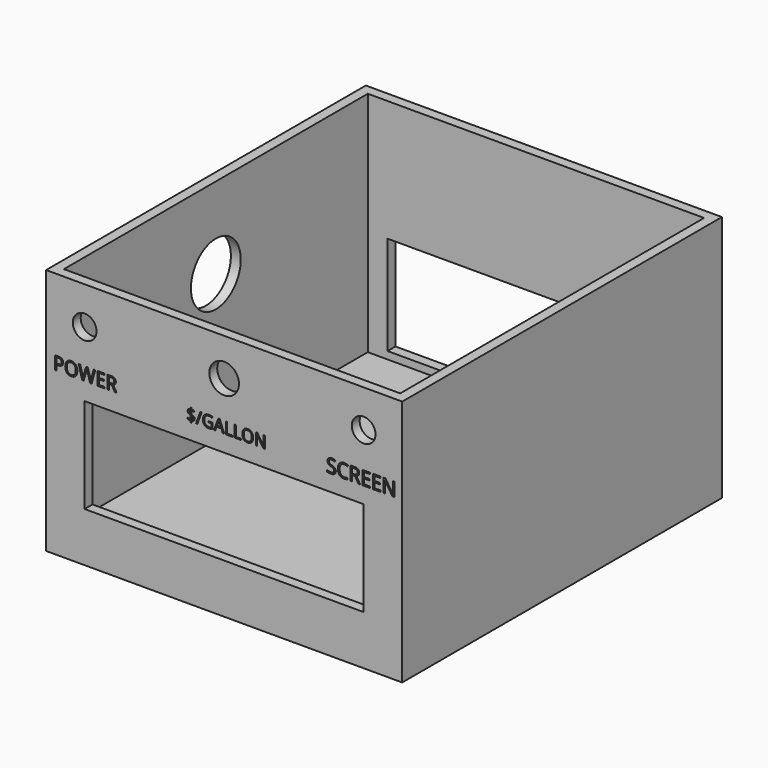
from build123d import *

# Parameters (mm, degrees)
F0_W          = 91.44
F0_H          = 102.616
F1_DEPTH      = 63.5
F2_W          = 86.36
F2_H          = 97.536
F3_DEPTH      = 58.42
F4_W          = 71.628
F4_H          = 24.384
F5_DEPTH      = 25.4
F6_R          = 3.048
F6_R_2        = 3.81
F7_DEPTH      = 7.62
F8_TEXT_SIZE  = 4.7196634114
F9_DEPTH      = 1.27
F10_TEXT_SIZE = 4.222859732
F11_DEPTH     = 1.27
F12_TEXT_SIZE = 4.8970176873
F13_DEPTH     = 1.27
F14_R         = 8.001
F15_DEPTH     = 7.62
F18_W         = 76.2
F18_H         = 25.4
F19_DEPTH     = 25.4


# Not quite as in the source:
# - Text() gives the source's letters only with a copy of the font that has no kerning and outlines rounded to 1/6400 em; it was checked with that copy


with BuildPart() as f1:
    # F0 (on Top) → F1 (new body)
    with BuildSketch(Plane.XY):
        Rectangle(F0_W, F0_H)
    extrude(amount=F1_DEPTH)

    # F2 (on face) → F3 (cut)
    with BuildSketch(Plane.XY.offset(63.5)):
        Rectangle(F2_W, F2_H)
    extrude(amount=-F3_DEPTH, mode=Mode.SUBTRACT)

    # F4 (on face) → F5 (cut)
    with BuildSketch(Plane.XZ.offset(51.308)):
        with Locations((0, 24.892)):
            Rectangle(F4_W, F4_H)
    extrude(amount=-F5_DEPTH, mode=Mode.SUBTRACT)

    # F6 (on face) → F7 (cut)
    with BuildSketch(Plane.XZ.offset(51.308)):
        with Locations((-35.814, 53.848)):
            Circle(F6_R)
        with Locations((0, 53.848)):
            Circle(F6_R_2)
        with Locations((35.814, 53.848)):
            Circle(F6_R)
    extrude(amount=-F7_DEPTH, mode=Mode.SUBTRACT)

    # F8 (on face) → F9 (cut)
    with BuildSketch(Plane.XZ.offset(51.308)):
        with Locations((-43.9296253026, 41.6202954948)):
            Text('POWER', F8_TEXT_SIZE, font='Open Sans', text_align=(TextAlign.LEFT, TextAlign.BOTTOM))
    extrude(amount=-F9_DEPTH, mode=Mode.SUBTRACT)

    # F10 (on face) → F11 (cut)
    with BuildSketch(Plane.XZ.offset(51.308)):
        with Locations((-9.6798079903, 41.3448065519)):
            Text('$/GALLON', F10_TEXT_SIZE, font='Open Sans', text_align=(TextAlign.LEFT, TextAlign.BOTTOM))
    extrude(amount=-F11_DEPTH, mode=Mode.SUBTRACT)

    # F12 (on face) → F13 (cut)
    with BuildSketch(Plane.XZ.offset(51.308)):
        with Locations((26.2173635299, 41.2667466118)):
            Text('SCREEN', F12_TEXT_SIZE, font='Open Sans', text_align=(TextAlign.LEFT, TextAlign.BOTTOM))
    extrude(amount=-F13_DEPTH, mode=Mode.SUBTRACT)

    # F14 (on face) → F15 (cut)
    with BuildSketch(Plane(origin=(-45.72, 0, 0), x_dir=(0, -1, 0), z_dir=(-1, 0, 0))):
        with Locations((0, 42.5877347589)):
            Circle(F14_R)
    extrude(amount=-F15_DEPTH, mode=Mode.SUBTRACT)

    # F18 (on face) → F19 (cut)
    with BuildSketch(Plane(origin=(0, 51.308, 0), x_dir=(-1, 0, 0), z_dir=(0, 1, 0))):
        with Locations((0, 19.688970819)):
            Rectangle(F18_W, F18_H)
    extrude(amount=-F19_DEPTH, mode=Mode.SUBTRACT)


solid = f1.part
